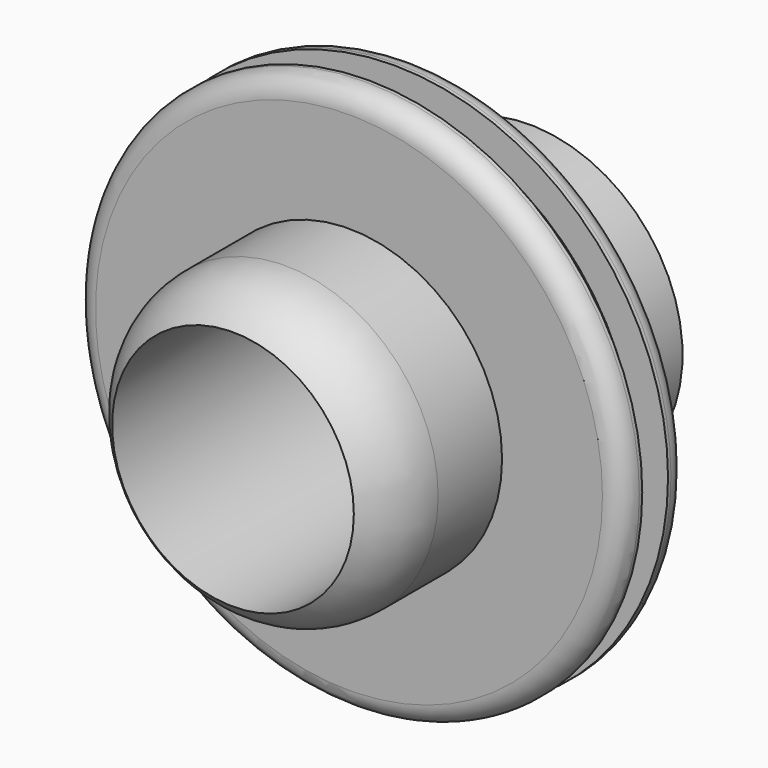
from build123d import *

# Parameters (mm, degrees)
F0_R      = 15
F1_DEPTH  = 2
F2_R      = 17
F2_R_2    = 15
F3_DEPTH  = 1.5
F4_R      = 17
F4_R_2    = 15
F5_DEPTH  = 1.5
F6_R      = 1.27
F7_R      = 9.5
F8_DEPTH  = 9
F9_R      = 9.5
F10_DEPTH = 9
F11_R     = 7.5
F12_DEPTH = 22
F13_R     = 0.762


# Not quite as in the source:
# - a fillet or chamfer that OpenCascade refuses, or shapes differently, is made with other operations: its cross-section is extruded or revolved along the edge and cut away or added
# - a pattern or mirror of a feature is missing from the dataset's text; its kind, count and spacing are read off the source's solid


with BuildPart() as f1:
    # F0 (on Front) → F1 (new body)
    with BuildSketch(Plane.XZ):
        Circle(F0_R)
    extrude(amount=F1_DEPTH)

    # F2 (on face) → F3 (join)
    with BuildSketch(Plane.XZ.offset(2)):
        Circle(F2_R)
        Circle(F2_R_2, mode=Mode.SUBTRACT)
        Circle(F2_R_2)
    f3 = extrude(amount=F3_DEPTH)

    # F3_copies: F3 across plane
    add(f3.mirror(Plane.ZX.offset(-1)))

    # F4 (on face) → F5 (join)
    with BuildSketch(Plane(origin=(0, 0, 0), x_dir=(-1, 0, 0), z_dir=(0, 1, 0))):
        Circle(F4_R)
        Circle(F4_R_2, mode=Mode.SUBTRACT)
    extrude(amount=F5_DEPTH)

    # F6
    f6_edges = [f1.edges().sort_by_distance(p)[0] for p in [
        (-17, -3.5, 0),
        (-17, 1.5, 0),
    ]]
    fillet(f6_edges, radius=F6_R)

    # F7 (on face) → F8 (join)
    with BuildSketch(Plane.XZ.offset(3.5)):
        Circle(F7_R)
    extrude(amount=F8_DEPTH)

    # F9 (on face) → F10 (join)
    with BuildSketch(Plane(origin=(0, 1.5, 0), x_dir=(-1, 0, 0), z_dir=(0, 1, 0))):
        Circle(F9_R)
    extrude(amount=F10_DEPTH)

    # F11 (on face) → F12 (cut)
    with BuildSketch(Plane.XZ.offset(12.5)):
        Circle(F11_R)
    extrude(amount=-F12_DEPTH, mode=Mode.SUBTRACT)

    # F13
    f13_edges = [f1.edges().sort_by_distance(p)[0] for p in [
        (-7.5, 9.5, 0),
    ]]
    fillet(f13_edges, radius=F13_R)

    # F14: fillet of radius 5.08 on 1 edges, made by hand

    # F14_s1 → F14_t2 (revolve, cut)
    with BuildSketch(Plane.XY):
        with BuildLine():
            ThreePointArc((7.5, -12.5), (8.9726256161, -10.7140835586), (9.5, -8.4601980247))
            Line((9.5, -8.4601980247), (9.5, -12.5))
            Line((9.5, -12.5), (7.5, -12.5))
        make_face()
    revolve(axis=Axis((0, -12.5, 0), (0, -1, 0)), mode=Mode.SUBTRACT)


solid = f1.part
